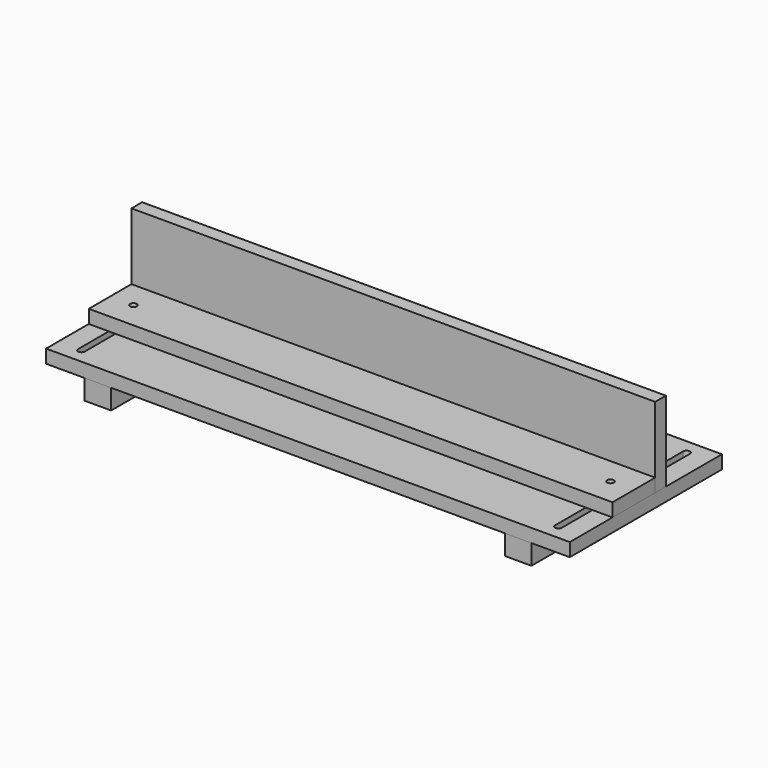
from build123d import *

# Parameters (mm, degrees)
F0_W      = 498.475
F0_H      = 180.975
F1_DEPTH  = 12.7
F2_W      = 25.4
F2_H      = 19.05
F3_DEPTH  = 180.975
F5_R      = 12.7
F6_DEPTH  = 25.4
F7_R      = 50.8
F8_DEPTH  = 6.35
F10_DEPTH = 25.4
F11_W     = 50.8
F11_H     = 12.7
F12_DEPTH = 249.2375
F13_R     = 3.175
F14_DEPTH = 25.4
F15_W     = 12.7
F15_H     = 76.2
F16_DEPTH = 249.2375


# Not quite as in the source:
# - a pattern or mirror of a feature is missing from the dataset's text; its kind, count and spacing are read off the source's solid


with BuildPart() as f1:
    # F0 (on Top) → F1 (new body)
    with BuildSketch(Plane.XY):
        Rectangle(F0_W, F0_H)
    extrude(amount=F1_DEPTH)

    # F5 (on face) → F6 (cut)
    with BuildSketch(Plane.XY.offset(12.7)):
        Circle(F5_R)
    extrude(amount=-F6_DEPTH, mode=Mode.SUBTRACT)

    # F7 (on face) → F8 (cut)
    with BuildSketch(Plane(origin=(0, 0, 0), x_dir=(1, 0, 0), z_dir=(0, 0, -1))):
        Circle(F7_R)
    extrude(amount=-F8_DEPTH, mode=Mode.SUBTRACT)

    # F9 (on face) → F10 (cut)
    with BuildSketch(Plane.XY.offset(12.7)):
        with BuildLine():
            Line((-230.1875, 76.2), (-230.1875, -76.2))
            ThreePointArc((-230.1875, -76.2), (-227.0125, -79.375), (-223.8375, -76.2))
            Line((-223.8375, -76.2), (-223.8375, 76.2))
            ThreePointArc((-223.8375, 76.2), (-227.0125, 79.375), (-230.1875, 76.2))
        make_face()
    f10 = extrude(amount=-F10_DEPTH, mode=Mode.SUBTRACT)

    # F10_copies: F10 across plane
    add(f10.mirror(Plane(origin=(0, 0, 0), x_dir=(0, 0, 1), z_dir=(1, 0, 0))), mode=Mode.SUBTRACT)


with BuildPart() as f3:
    # F2 (on face) → F3 (new body, through all)
    with BuildSketch(Plane.XZ.offset(90.4875)):
        with Locations((-200.025, -9.525)):
            Rectangle(F2_W, F2_H)
    extrude(amount=-F3_DEPTH)


with BuildPart() as f4_1:
    # F4: instance of F3
    add(f3.part.mirror(Plane.YZ))


with BuildPart() as f12:
    # F11 (on Right) → F12 (new body, symmetric)
    with BuildSketch(Plane.YZ):
        with Locations((-14.2875, 19.05)):
            Rectangle(F11_W, F11_H)
    extrude(amount=F12_DEPTH, both=True)

    # F13 (on face) → F14 (cut)
    with BuildSketch(Plane.XY.offset(25.4)):
        with Locations((-227.0125, -14.2875)):
            Circle(F13_R)
    f14 = extrude(amount=-F14_DEPTH, mode=Mode.SUBTRACT)

    # F14_copies: F14 across plane
    add(f14.mirror(Plane(origin=(0, 0, 0), x_dir=(0, 0, 1), z_dir=(1, 0, 0))), mode=Mode.SUBTRACT)


with BuildPart() as f16:
    # F15 (on Right) → F16 (new body, symmetric)
    with BuildSketch(Plane.YZ):
        with Locations((17.4625, 50.8)):
            Rectangle(F15_W, F15_H)
    extrude(amount=F16_DEPTH, both=True)


solid = Compound([f1.part, f3.part, f4_1.part, f12.part, f16.part])
